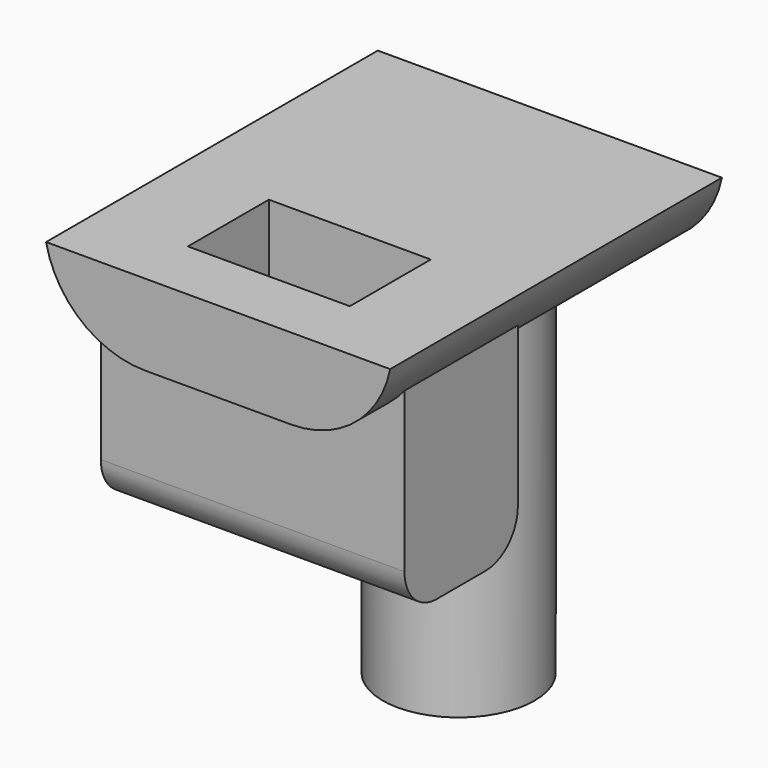
from build123d import *

# Parameters (mm, degrees)
F1_W         = 8.5
F1_H         = 20.4836754128
F2_DEPTH     = 4
F3_DEPTH     = 12
F4_DEPTH     = 4
F5_DEPTH     = 10
F6_T1_DEPTH  = 25
F7_T4_DEPTH  = 44.9785728407
F7_S6_R      = 3.75
F7_T7_DEPTH  = 24
F7_T11_DEPTH = 44.9785728407
F7_T16_DEPTH = 44.9785728407
F7_T21_DEPTH = 44.9785728407
F7_T26_DEPTH = 44.9785728407
F7_T31_DEPTH = 44.9785728407
F7_S33_R     = 3.75
F7_T34_DEPTH = 24


# Not quite as in the source:
# - a fillet or chamfer that OpenCascade refuses, or shapes differently, is made with other operations: its cross-section is extruded or revolved along the edge and cut away or added


with BuildPart() as f2:
    # F1 (on Top) → F2 (new body)
    with BuildSketch(Plane.XY):
        with Locations((4.25, -4.6106860973)):
            Rectangle(F1_W, F1_H)
        with Locations((-4.25, -4.6106860973)):
            Rectangle(F1_W, F1_H)
    extrude(amount=-F2_DEPTH)

    # F0 (on Top) → F3 (join)
    with BuildSketch(Plane.XY):
        with BuildLine():
            ThreePointArc((3.75, 0), (-2.6516504294, 2.6516504294), (0, -3.75))
            ThreePointArc((0, -3.75), (2.6516504294, -2.6516504294), (3.75, 0))
        make_face()
        with BuildLine():
            ThreePointArc((0, -2.25), (-1.5909902577, 1.5909902577), (2.25, 0))
            ThreePointArc((2.25, 0), (1.5909902577, -1.5909902577), (0, -2.25))
        make_face(mode=Mode.SUBTRACT)
        Polygon((7.5, -5.7213721946), (0, -5.7213721946), (-7.5, -5.7213721946), (-7.5, -12.7213721946), (7.5, -12.7213721946), align=None)
        Polygon((-4, -6.7213721946), (0, -6.7213721946), (4, -6.7213721946), (4, -11.7213721946), (-4, -11.7213721946), align=None, mode=Mode.SUBTRACT)
    extrude(amount=-F3_DEPTH)

    # F4 (cut): a face of the model
    f4_faces = [f2.faces().sort_by_distance(p)[0] for p in [
        (0, -9.2213721946, -4),
    ]]
    extrude(f4_faces, amount=-F4_DEPTH, mode=Mode.SUBTRACT)

    # F5 (add): a face of the model
    f5_faces = [f2.faces().sort_by_distance(p)[0] for p in [
        (0, 3.6439339828, -12),
    ]]
    extrude(f5_faces, amount=F5_DEPTH)

    # F6: fillet of radius 2 on 2 edges, made by hand

    # F6_s2 → F6_t1 (cut)
    with BuildSketch(Plane.YZ.offset(-12.5)):
        with BuildLine():
            ThreePointArc((-10.7213721946, -12), (-12.135585757, -11.4142135624), (-12.7213721946, -10))
            Line((-12.7213721946, -10), (-12.7213721946, -12))
            Line((-12.7213721946, -12), (-10.7213721946, -12))
        make_face()
        with BuildLine():
            ThreePointArc((-7.7213721946, -12), (-6.3071586322, -11.4142135624), (-5.7213721946, -10))
            Line((-5.7213721946, -10), (-5.7213721946, -12))
            Line((-5.7213721946, -12), (-7.7213721946, -12))
        make_face()
    extrude(amount=F6_T1_DEPTH, mode=Mode.SUBTRACT)

    # F7: fillet of radius 5 on 2 edges, made by hand


with BuildPart() as f7_tool2:
    # F7_s3 → F7_t4 (new body)
    with BuildSketch(Plane.XZ.offset(-17.8786003231)):
        with BuildLine():
            ThreePointArc((-3.6010205144, -4), (-6.7632981746, -2.8729833462), (-8.5, 0))
            Line((-8.5, 0), (-8.5, -4))
            Line((-8.5, -4), (-3.6010205144, -4))
        make_face()
    extrude(amount=F7_T4_DEPTH)

    split(bisect_by=Plane.XZ.offset(5.7213721946), keep=Keep.BOTTOM)

    # F7_s6 → F7_t7 (cut, symmetric)
    with BuildSketch(Plane.XY.offset(-2)):
        Circle(F7_S6_R)
    extrude(amount=F7_T7_DEPTH, both=True, mode=Mode.SUBTRACT)


with BuildPart() as f2_1:
    add(f2.part)

    # F7_t1: cut F7_tool2
    add(f7_tool2.part, mode=Mode.SUBTRACT)


with BuildPart() as f7_tool9:
    # F7_s10 → F7_t11 (new body)
    with BuildSketch(Plane.XZ.offset(-17.8786003231)):
        with BuildLine():
            ThreePointArc((-3.6010205144, -4), (-6.7632981746, -2.8729833462), (-8.5, 0))
            Line((-8.5, 0), (-8.5, -4))
            Line((-8.5, -4), (-3.6010205144, -4))
        make_face()
    extrude(amount=F7_T11_DEPTH)

    split(bisect_by=Plane.YZ.offset(-7.5), keep=Keep.BOTTOM)


with BuildPart() as f2_2:
    add(f2_1.part)

    # F7_t8: cut F7_tool9
    add(f7_tool9.part, mode=Mode.SUBTRACT)


with BuildPart() as f7_tool14:
    # F7_s15 → F7_t16 (new body)
    with BuildSketch(Plane.XZ.offset(-17.8786003231)):
        with BuildLine():
            ThreePointArc((-3.6010205144, -4), (-6.7632981746, -2.8729833462), (-8.5, 0))
            Line((-8.5, 0), (-8.5, -4))
            Line((-8.5, -4), (-3.6010205144, -4))
        make_face()
    extrude(amount=F7_T16_DEPTH)

    split(bisect_by=Plane.XZ.offset(12.7213721946), keep=Keep.TOP)


with BuildPart() as f2_3:
    add(f2_2.part)

    # F7_t13: cut F7_tool14
    add(f7_tool14.part, mode=Mode.SUBTRACT)


with BuildPart() as f7_tool19:
    # F7_s20 → F7_t21 (new body)
    with BuildSketch(Plane.XZ.offset(27.0999725176)):
        with BuildLine():
            ThreePointArc((8.5, 0), (6.7632981746, -2.8729833462), (3.6010205144, -4))
            Line((3.6010205144, -4), (8.5, -4))
            Line((8.5, -4), (8.5, 0))
        make_face()
    extrude(amount=-F7_T21_DEPTH)

    split(bisect_by=Plane.YZ.offset(7.5), keep=Keep.TOP)


with BuildPart() as f2_4:
    add(f2_3.part)

    # F7_t18: cut F7_tool19
    add(f7_tool19.part, mode=Mode.SUBTRACT)


with BuildPart() as f7_tool24:
    # F7_s25 → F7_t26 (new body)
    with BuildSketch(Plane.XZ.offset(27.0999725176)):
        with BuildLine():
            ThreePointArc((8.5, 0), (6.7632981746, -2.8729833462), (3.6010205144, -4))
            Line((3.6010205144, -4), (8.5, -4))
            Line((8.5, -4), (8.5, 0))
        make_face()
    extrude(amount=-F7_T26_DEPTH)

    split(bisect_by=Plane.XZ.offset(12.7213721946), keep=Keep.TOP)


with BuildPart() as f2_5:
    add(f2_4.part)

    # F7_t23: cut F7_tool24
    add(f7_tool24.part, mode=Mode.SUBTRACT)


with BuildPart() as f7_tool29:
    # F7_s30 → F7_t31 (new body)
    with BuildSketch(Plane.XZ.offset(27.0999725176)):
        with BuildLine():
            ThreePointArc((8.5, 0), (6.7632981746, -2.8729833462), (3.6010205144, -4))
            Line((3.6010205144, -4), (8.5, -4))
            Line((8.5, -4), (8.5, 0))
        make_face()
    extrude(amount=-F7_T31_DEPTH)

    split(bisect_by=Plane.XZ.offset(5.7213721946), keep=Keep.BOTTOM)

    # F7_s33 → F7_t34 (cut, symmetric)
    with BuildSketch(Plane.XY.offset(-2)):
        Circle(F7_S33_R)
    extrude(amount=F7_T34_DEPTH, both=True, mode=Mode.SUBTRACT)


with BuildPart() as f2_6:
    add(f2_5.part)

    # F7_t28: cut F7_tool29
    add(f7_tool29.part, mode=Mode.SUBTRACT)


solid = f2_6.part
